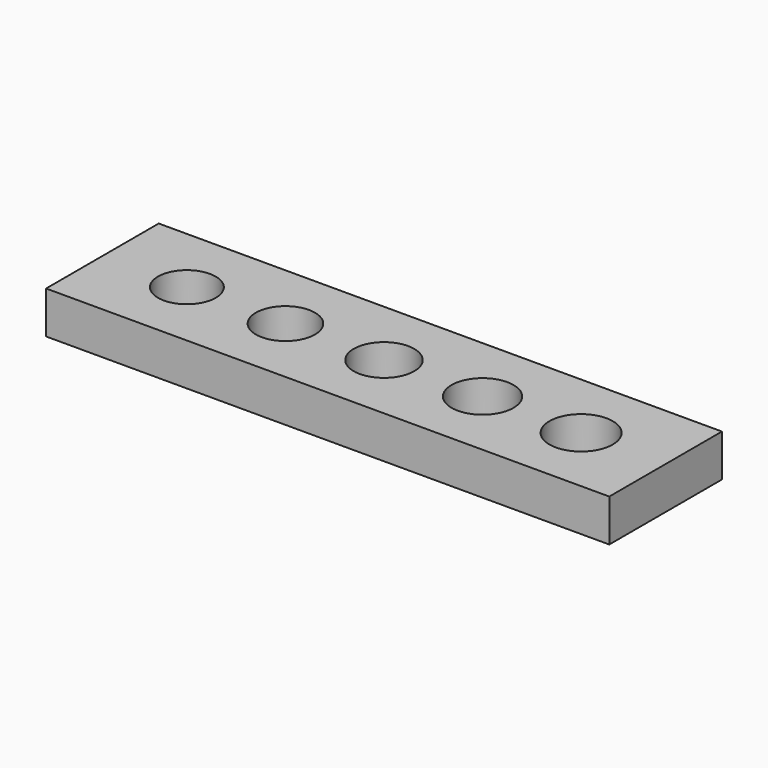
from build123d import *

# Parameters (mm, degrees)
F0_W     = 40
F0_H     = 10
F0_R     = 2.05
F0_R_2   = 2.1
F0_R_3   = 2.15
F0_R_4   = 2.2
F0_R_5   = 2.25
F1_DEPTH = 3


# Not quite as in the source:
# - a feature of the source that left no trace in its solid (it failed there, or was rolled back) is left out


with BuildPart() as f1:
    # F0 (on Top) → F1 (new body)
    with BuildSketch(Plane.XY):
        Rectangle(F0_W, F0_H)
        with Locations((-14, 0)):
            Circle(F0_R, mode=Mode.SUBTRACT)
        with Locations((-7, 0)):
            Circle(F0_R_2, mode=Mode.SUBTRACT)
        Circle(F0_R_3, mode=Mode.SUBTRACT)
        with Locations((7, 0)):
            Circle(F0_R_4, mode=Mode.SUBTRACT)
        with Locations((14, 0)):
            Circle(F0_R_5, mode=Mode.SUBTRACT)
    extrude(amount=F1_DEPTH)


solid = f1.part
